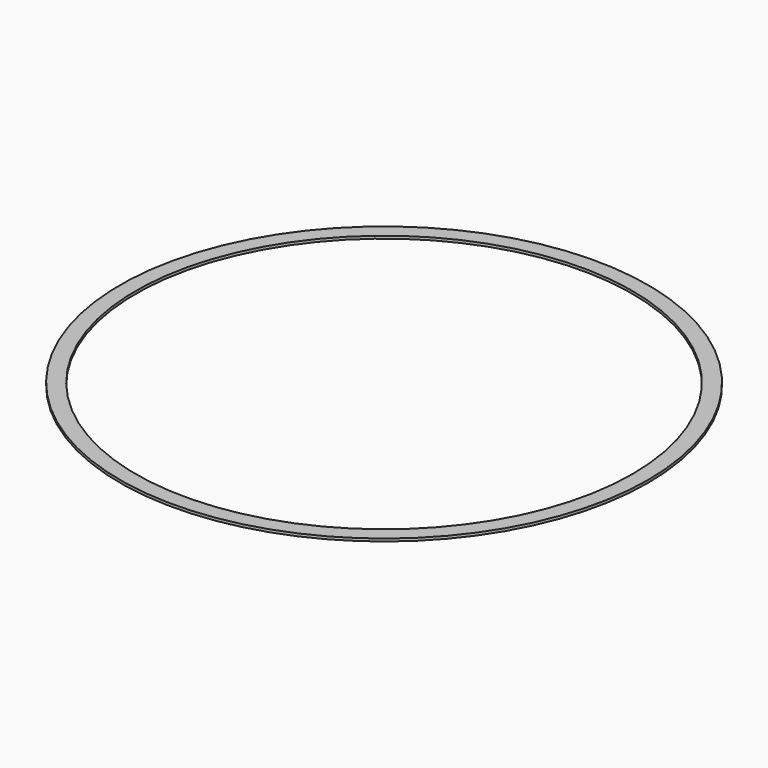
from build123d import *

# Parameters (mm, degrees)
F0_R     = 426.24502
F0_R_2   = 400.84502
F1_DEPTH = 4.2333333333


# Not quite as in the source:
# - a length typed as a fraction of an inch, garbled in the dataset ("3 / 203.2 mm" for 3/8 in), is restored


with BuildPart() as f1:
    # F0 (on Top) → F1 (new body)
    with BuildSketch(Plane.XY):
        Circle(F0_R)
        Circle(F0_R_2, mode=Mode.SUBTRACT)
    extrude(amount=F1_DEPTH)


solid = f1.part
